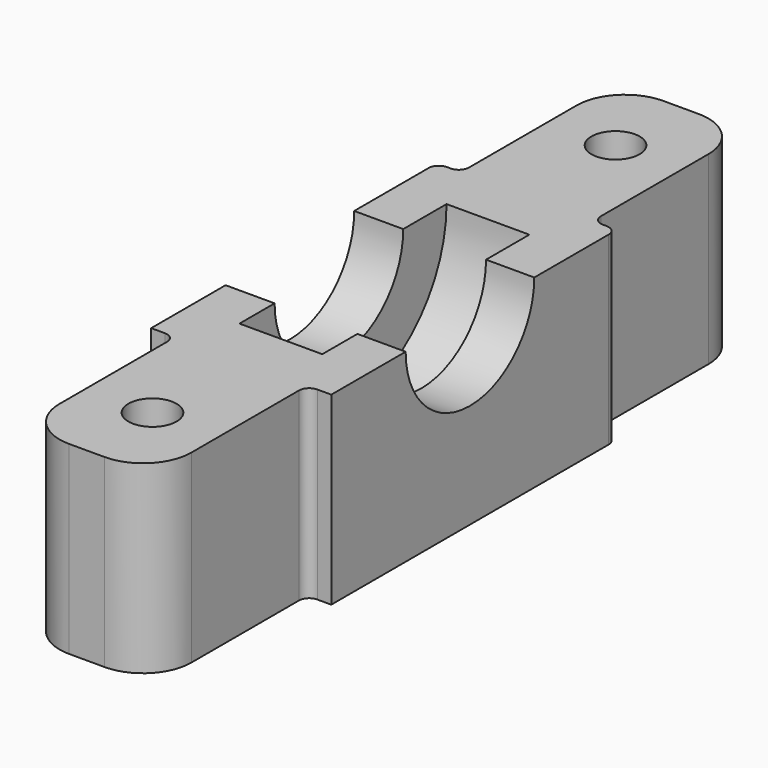
from build123d import *

# Parameters (mm, degrees)
F0_R     = 1.5
F0_W     = 5.1
F0_H     = 16.1
F1_DEPTH = 11.5
F3_DEPTH = 25


# Not quite as in the source:
# - a feature names something its author has since deleted; it is built from what else it names


with BuildPart() as f1:
    # F0 (on Top) → F1 (new body)
    with BuildSketch(Plane.XY):
        with BuildLine():
            ThreePointArc((5.5999997705, 10.465261464), (5.4140892248, 10.9140892248), (4.965261464, 11.0999997705))
            Line((4.965261464, 11.0999997705), (4.734738077, 11.0999997705))
            Line((4.734738077, 11.0999997705), (-4.734738077, 11.0999997705))
            Line((-4.734738077, 11.0999997705), (-4.965261464, 11.0999997705))
            ThreePointArc((-4.965261464, 11.0999997705), (-5.4140892248, 10.9140892248), (-5.5999997705, 10.465261464))
            Line((-5.5999997705, 10.465261464), (-5.5999997705, -10.465261464))
            ThreePointArc((-5.5999997705, -10.465261464), (-5.4140892248, -10.9140892248), (-4.965261464, -11.0999997705))
            Line((-4.965261464, -11.0999997705), (-4.734738077, -11.0999997705))
            Line((-4.734738077, -11.0999997705), (4.734738077, -11.0999997705))
            Line((4.734738077, -11.0999997705), (4.965261464, -11.0999997705))
            ThreePointArc((4.965261464, -11.0999997705), (5.4140892248, -10.9140892248), (5.5999997705, -10.465261464))
            Line((5.5999997705, -10.465261464), (5.5999997705, 10.465261464))
        make_face()
        Polygon((2.6, 8.1), (2.6, 0), (2.6, -8.1), (-2.6, -8.1), (-2.6, 8.1), align=None, mode=Mode.SUBTRACT)
        with BuildLine():
            Line((-4.734738077, 11.0999997705), (4.734738077, 11.0999997705))
            ThreePointArc((4.734738077, 11.0999997705), (4.2859103162, 11.2859103162), (4.0999997705, 11.734738077))
            Line((4.0999997705, 11.734738077), (4.0999997705, 20.0999997705))
            ThreePointArc((4.0999997705, 20.0999997705), (3.2213201141, 22.2213201141), (1.0999997705, 23.0999997705))
            Line((1.0999997705, 23.0999997705), (-1.0999997705, 23.0999997705))
            ThreePointArc((-1.0999997705, 23.0999997705), (-3.2213201141, 22.2213201141), (-4.0999997705, 20.0999997705))
            Line((-4.0999997705, 20.0999997705), (-4.0999997705, 11.734738077))
            ThreePointArc((-4.0999997705, 11.734738077), (-4.2859103162, 11.2859103162), (-4.734738077, 11.0999997705))
        make_face()
        with Locations((0, 18)):
            Circle(F0_R, mode=Mode.SUBTRACT)
        with BuildLine():
            ThreePointArc((4.0999997705, -11.734738077), (4.2859103162, -11.2859103162), (4.734738077, -11.0999997705))
            Line((4.734738077, -11.0999997705), (-4.734738077, -11.0999997705))
            ThreePointArc((-4.734738077, -11.0999997705), (-4.2859103162, -11.2859103162), (-4.0999997705, -11.734738077))
            Line((-4.0999997705, -11.734738077), (-4.0999997705, -20.0999997705))
            ThreePointArc((-4.0999997705, -20.0999997705), (-3.2213201141, -22.2213201141), (-1.0999997705, -23.0999997705))
            Line((-1.0999997705, -23.0999997705), (1.0999997705, -23.0999997705))
            ThreePointArc((1.0999997705, -23.0999997705), (3.2213201141, -22.2213201141), (4.0999997705, -20.0999997705))
            Line((4.0999997705, -20.0999997705), (4.0999997705, -11.734738077))
        make_face()
        with Locations((0, -18)):
            Circle(F0_R, mode=Mode.SUBTRACT)
        Polygon((2.6, -8.1), (2.6, 0), (2.6, 8.1), (-2.6, 8.1), (-2.6, -8.1), align=None)
        Rectangle(F0_W, F0_H, mode=Mode.SUBTRACT)
        Rectangle(F0_W, F0_H)
        with BuildLine():
            Line((5.5999997705, -11.0999997705), (5.5999997705, -10.465261464))
            ThreePointArc((5.5999997705, -10.465261464), (5.4140892248, -10.9140892248), (4.965261464, -11.0999997705))
            Line((4.965261464, -11.0999997705), (5.5999997705, -11.0999997705))
        make_face()
        with BuildLine():
            ThreePointArc((-4.965261464, -11.0999997705), (-5.4140892248, -10.9140892248), (-5.5999997705, -10.465261464))
            Line((-5.5999997705, -10.465261464), (-5.5999997705, -11.0999997705))
            Line((-5.5999997705, -11.0999997705), (-4.965261464, -11.0999997705))
        make_face()
    extrude(amount=F1_DEPTH)

    # F2 (on face) → F3 (cut)
    with BuildSketch(Plane.YZ.offset(5.5999997705)):
        with BuildLine():
            ThreePointArc((-5.3173691533, 11.5), (-0.3173691533, 6.5), (4.6826308467, 11.5))
            Line((4.6826308467, 11.5), (-5.3173691533, 11.5))
        make_face()
    extrude(amount=-F3_DEPTH, mode=Mode.SUBTRACT)

    # F4 (on face) → F5 (revolve, cut)
    with BuildSketch(Plane.XY.offset(11.5)):
        Polygon((2.55, 8.05), (-2.55, 8.05), (-2.55, 4.6826308467), (2.6, 4.6826308467), (2.6, 8.05), align=None)
        Polygon((2.6, 4.6826308467), (-2.55, 4.6826308467), (-2.55, 0), (0, 0), (2.6, 0), align=None)
    revolve(axis=Axis((0.025, 0, 11.5), (-1, 0, 0)), mode=Mode.SUBTRACT)


solid = f1.part
